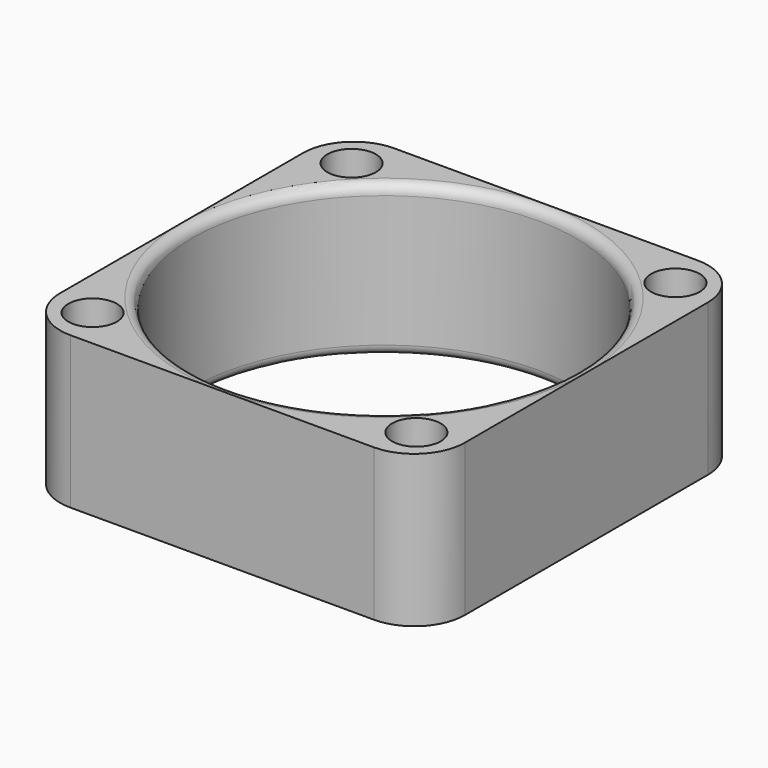
from build123d import *

# Parameters (mm, degrees)
F0_W     = 40
F0_H     = 40
F0_R     = 2.4
F0_R_2   = 19
F1_DEPTH = 15
F2_R     = 5
F3_R     = 0.99999


# Not quite as in the source:
# - a fillet or chamfer is up to 0.001 mm smaller than in the source, because OpenCascade refuses the exact size


with BuildPart() as f1:
    # F0 (on Top) → F1 (new body)
    with BuildSketch(Plane.XY):
        Rectangle(F0_W, F0_H)
        with Locations((-16, -16)):
            Circle(F0_R, mode=Mode.SUBTRACT)
        with Locations((16, -16)):
            Circle(F0_R, mode=Mode.SUBTRACT)
        with Locations((-16, 16)):
            Circle(F0_R, mode=Mode.SUBTRACT)
        Circle(F0_R_2, mode=Mode.SUBTRACT)
        with Locations((16, 16)):
            Circle(F0_R, mode=Mode.SUBTRACT)
    extrude(amount=F1_DEPTH)

    # F2
    f2_edges = [f1.edges().sort_by_distance(p)[0] for p in [
        (20, 20, 7.5),
        (20, -20, 7.5),
        (-20, 20, 7.5),
        (-20, -20, 7.5),
    ]]
    fillet(f2_edges, radius=F2_R)

    # F3 (radius 1 in the source; OpenCascade refuses exactly that, so slightly less here)
    f3_edges = [f1.edges().sort_by_distance(p)[0] for p in [
        (-19, 0, 15),
        (-19, 0, 0),
    ]]
    fillet(f3_edges, radius=F3_R)


solid = f1.part
